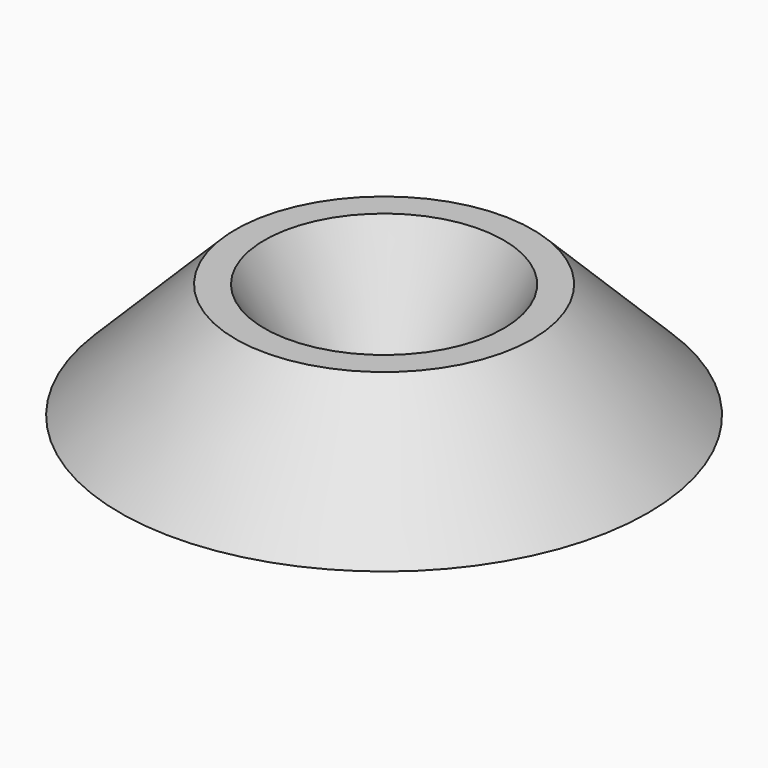
from build123d import *

# Parameters (mm, degrees)
F0_R     = 8
F1_DEPTH = 3.5
F2_SIZE  = 3.49999
F3_R     = 3.625
F4_R     = 1.625


# Not quite as in the source:
# - a fillet or chamfer is up to 0.001 mm smaller than in the source, because OpenCascade refuses the exact size


with BuildPart() as f1:
    # F0 (on Top) → F1 (new body)
    with BuildSketch(Plane.XY):
        Circle(F0_R)
    extrude(amount=F1_DEPTH)

    # F2 (size 3.5 in the source; OpenCascade refuses exactly that, so slightly less here)
    f2_edges = [f1.edges().sort_by_distance(p)[0] for p in [
        (-8, 0, 3.5),
    ]]
    chamfer(f2_edges, length=F2_SIZE)

    # F3 (on face) → F5 section 0
    with BuildSketch(Plane.XY.offset(3.5)):
        Circle(F3_R)
    # F4 (on Top) → F5 section 1
    with BuildSketch(Plane.XY):
        Circle(F4_R)
    loft(mode=Mode.SUBTRACT)


solid = f1.part
